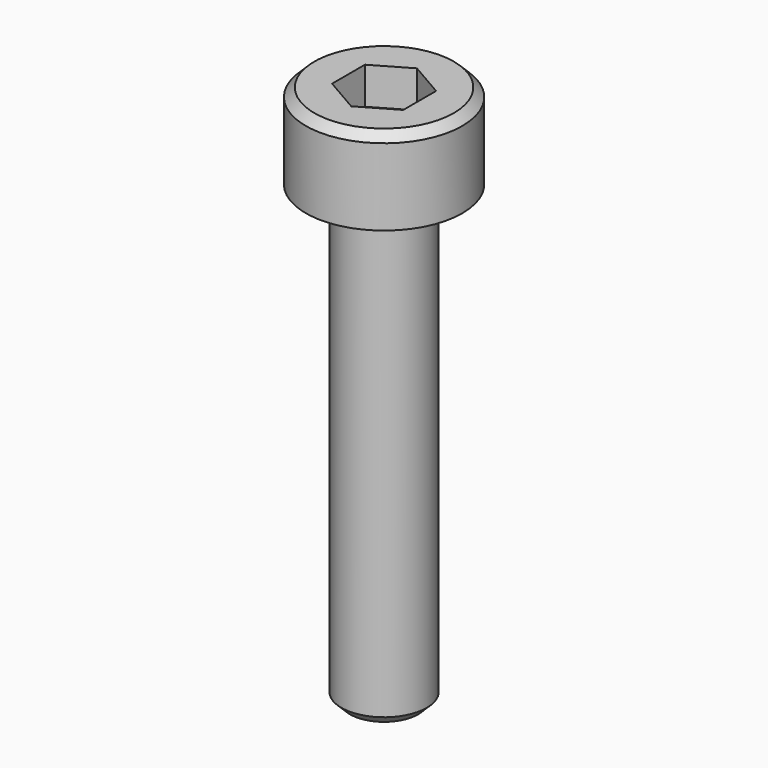
from build123d import *

# Parameters (mm, degrees)
F2_R      = 1.5
F3_DEPTH  = 16
F2_R_2    = 2.75
F3_FACE_R = 1.5
F4_DEPTH  = 3
F5_SIZE   = 0.3
F7_DEPTH  = 1.3


with BuildPart() as f3:
    # F2 (on Top) → F3 (new body)
    with BuildSketch(Plane.XY):
        Circle(F2_R)
    extrude(amount=-F3_DEPTH)

    # F2 (on Top) + F3_face (on face) → F4 (join)
    with BuildSketch(Plane.XY):
        Circle(F2_R_2)
        Circle(F2_R, mode=Mode.SUBTRACT)
    with BuildSketch(Plane.XY):
        Circle(F3_FACE_R)
    extrude(amount=F4_DEPTH)

    # F5
    f5_edges = [f3.edges().sort_by_distance(p)[0] for p in [
        (-1.5, 0, -16),
        (-2.75, 0, 3),
    ]]
    chamfer(f5_edges, length=F5_SIZE)

    # F6 (on face) → F7 (cut)
    with BuildSketch(Plane.XY.offset(3)):
        Polygon((1.25, -0.7216878365), (1.25, 0.7216878365), (0, 1.443375673), (-1.25, 0.7216878365), (-1.25, -0.7216878365), (0, -1.443375673), align=None)
    extrude(amount=-F7_DEPTH, mode=Mode.SUBTRACT)


solid = f3.part
